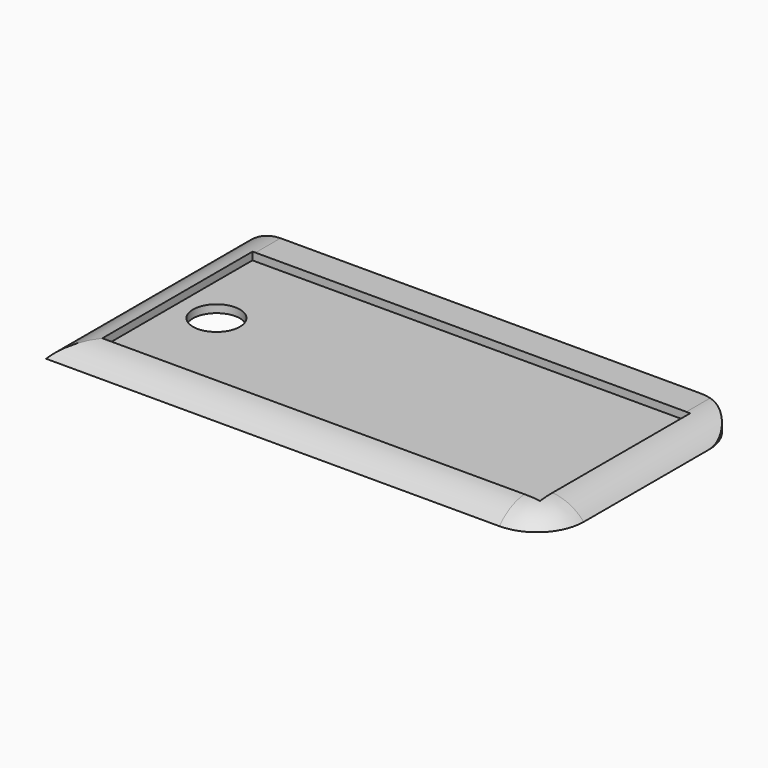
from build123d import *

# Parameters (mm, degrees)
F0_W        = 50.8
F0_H        = 25.4
F0_W_2      = 44.45
F0_H_2      = 19.05
F0_R        = 2.38125
F1_DEPTH    = 0.79375
F2_DEPTH    = 1.5875
F3_R        = 4.7625
F4_T1_DEPTH = 25.4
F4_T3_DEPTH = 54.9118947857
F4_T5_DEPTH = 29.5118947857
F4_T8_ANGLE = 90
F5_T1_DEPTH = 39.6011909767


# Not quite as in the source:
# - a fillet or chamfer that OpenCascade refuses, or shapes differently, is made with other operations: its cross-section is extruded or revolved along the edge and cut away or added


with BuildPart() as f1:
    # F0 (on Top) → F1 (new body)
    with BuildSketch(Plane.XY):
        with Locations((25.4, 12.7)):
            Rectangle(F0_W, F0_H)
        with Locations((25.4, 12.7)):
            Rectangle(F0_W_2, F0_H_2, mode=Mode.SUBTRACT)
        with Locations((25.4, 12.7)):
            Rectangle(F0_W_2, F0_H_2)
        with Locations((7.14375, 12.7)):
            Circle(F0_R, mode=Mode.SUBTRACT)
    extrude(amount=F1_DEPTH)

    # F0 (on Top) → F2 (join)
    with BuildSketch(Plane.XY):
        with Locations((25.4, 12.7)):
            Rectangle(F0_W, F0_H)
        with Locations((25.4, 12.7)):
            Rectangle(F0_W_2, F0_H_2, mode=Mode.SUBTRACT)
    extrude(amount=F2_DEPTH)

    # F3
    f3_edges = [f1.edges().sort_by_distance(p)[0] for p in [
        (50.8, 0, 0.79375),
    ]]
    fillet(f3_edges, radius=F3_R)

    # F4: fillet of radius 4.7625 on 2 edges, made by hand

    # F4_s2 → F4_t1 (cut)
    with BuildSketch(Plane.XY.offset(-11.90625)):
        with BuildLine():
            ThreePointArc((50.8, 20.6375), (49.4050960454, 24.0050960454), (46.0375, 25.4))
            Line((46.0375, 25.4), (50.8, 25.4))
            Line((50.8, 25.4), (50.8, 20.6375))
        make_face()
    extrude(amount=F4_T1_DEPTH, mode=Mode.SUBTRACT)

    # F4_s4 → F4_t3 (cut)
    with BuildSketch(Plane.YZ.offset(-8.8743947857)):
        with BuildLine():
            ThreePointArc((3.5497579143, 1.5875), (1.6054754309, 1.1725478002), (0, 0))
            Line((0, 0), (0, 1.5875))
            Line((0, 1.5875), (3.5497579143, 1.5875))
        make_face()
    extrude(amount=F4_T3_DEPTH, mode=Mode.SUBTRACT)

    # F4_s6 → F4_t5 (cut)
    with BuildSketch(Plane.XZ.offset(-34.2743947857)):
        with BuildLine():
            ThreePointArc((47.2502420857, 1.5875), (49.1945245691, 1.1725478002), (50.8, 0))
            Line((50.8, 0), (50.8, 1.5875))
            Line((50.8, 1.5875), (47.2502420857, 1.5875))
        make_face()
    extrude(amount=F4_T5_DEPTH, mode=Mode.SUBTRACT)

    # F4_s7 → F4_t8 (revolve, cut)
    with BuildSketch(Plane.XZ.offset(-4.7625)):
        with BuildLine():
            ThreePointArc((47.2502420857, 1.5875), (49.1945245691, 1.1725478002), (50.8, 0))
            Line((50.8, 0), (50.8, 1.5875))
            Line((50.8, 1.5875), (47.2502420857, 1.5875))
        make_face()
    revolve(axis=Axis((46.0375, 4.7625, 1.5875), (0, 0, -1)), revolution_arc=F4_T8_ANGLE, mode=Mode.SUBTRACT)

    # F5: fillet of radius 4.7625 on 1 edges, made by hand

    # F5_s2 → F5_t1 (cut)
    with BuildSketch(Plane.XZ.offset(-34.2754744455)):
        with BuildLine():
            ThreePointArc((-0.0002981182, 0.0002666937), (1.6055468798, 1.1729169704), (3.5501897557, 1.5879))
            Line((3.5501897557, 1.5879), (3.5501897557, 2.0642865685))
            ThreePointArc((3.5501897557, 2.0642865685), (1.7750948778, 2.0638865685), (0, 2.0638865685))
            Line((0, 2.0638865685), (-0.4763865685, 1.5875))
            ThreePointArc((-0.4763865685, 1.5875), (-0.4763865685, 0.7938833468), (-0.3553469056, 0.3178899316))
            Line((-0.3553469056, 0.3178899316), (-0.0002981182, 0.0002666937))
        make_face()
    extrude(amount=F5_T1_DEPTH, mode=Mode.SUBTRACT)


solid = f1.part
